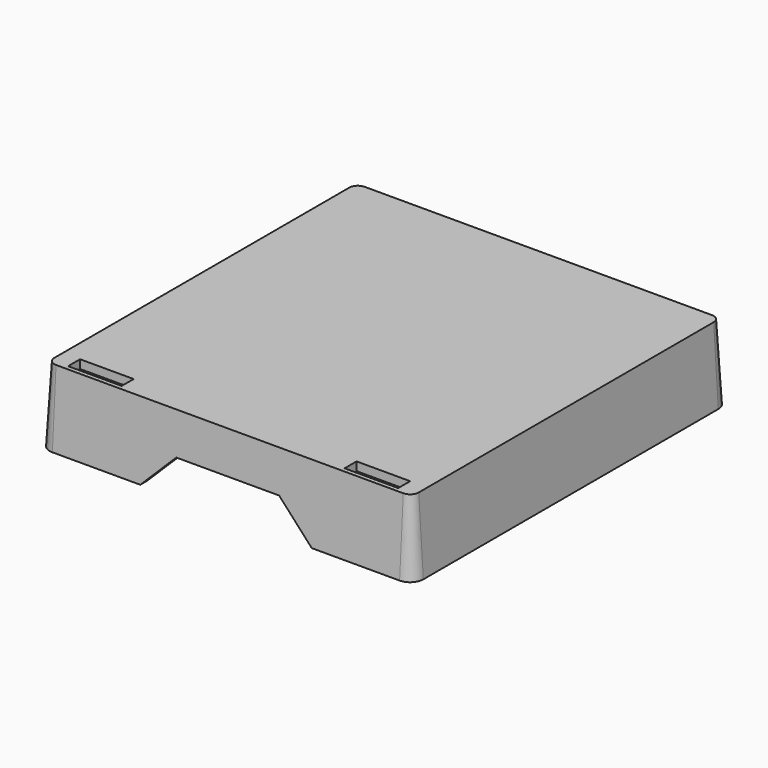
from build123d import *

# Parameters (mm, degrees)
F1_DEPTH  = 17.5
F1_TAPER  = -3.5
F3_DEPTH  = 75
F4_T      = 2
F5_W      = 12.5
F5_H      = 3.5
F6_DEPTH  = 17.5010001
F7_R      = 4
F8_DEPTH  = 31.5
F9_SIZE   = 3
F11_W     = 25
F11_H     = 20
F12_DEPTH = 10


# Not quite as in the source:
# - a shell that OpenCascade refuses in one call is made with other operations: the cavity is built on its own and cut out


with BuildPart() as f1:
    # F0 (on Top) → F1 (new body)
    with BuildSketch(Plane.XY):
        with BuildLine():
            Line((-40.5, -45), (40.5, -45))
            ThreePointArc((40.5, -45), (41.9142135624, -44.4142135624), (42.5, -43))
            Line((42.5, -43), (42.5, 43))
            ThreePointArc((42.5, 43), (41.9142135624, 44.4142135624), (40.5, 45))
            Line((40.5, 45), (-40.5, 45))
            ThreePointArc((-40.5, 45), (-41.9142135624, 44.4142135624), (-42.5, 43))
            Line((-42.5, 43), (-42.5, -43))
            ThreePointArc((-42.5, -43), (-41.9142135624, -44.4142135624), (-40.5, -45))
        make_face()
    extrude(amount=-F1_DEPTH, taper=F1_TAPER)

    # F2 (on Front) → F3 (cut, symmetric)
    with BuildSketch(Plane.XZ):
        Polygon((-20, -17.5), (0, -17.5), (20, -17.5), (12, -9.5), (0, -9.5), (-12, -9.5), align=None)
    extrude(amount=F3_DEPTH, both=True, mode=Mode.SUBTRACT)

    # F4: shell of thickness 2, made by hand


with BuildPart() as f4_core1:
    # F4_t2: copy of F1
    add(f1.part)

    # the walls: a layer under each face that stays
    f4_faces = [f4_core1.faces().sort_by_distance(p)[0] for p in [
        (0, -45.5351729263, -8.75),
        (-42.2926379677, -44.7926379677, -8.75),
        (42.2926379677, -44.7926379677, -8.75),
        (0, 0, 0),
        (-43.0351729263, 0, -8.75),
        (-42.2926379677, 44.7926379677, -8.75),
        (0, 45.5351729263, -8.75),
        (42.2926379677, 44.7926379677, -8.75),
        (43.0351729263, 0, -8.75),
    ]]
    thicken(f4_faces, amount=-F4_T, mode=Mode.SUBTRACT)


with BuildPart() as f1_1:
    add(f1.part)

    # what is left inside the walls is the cavity
    f4_cavity = [f4_core1.part.solids().sort_by_distance(p)[0] for p in [
        (-13.539529, 0, -2.02),
    ]]
    add(f4_cavity, mode=Mode.SUBTRACT)

    # F5 (on Top) → F6 (cut, through all)
    with BuildSketch(Plane.XY):
        with Locations((-32.25, -42.25)):
            Rectangle(F5_W, F5_H)
        with Locations((32.25, -42.25)):
            Rectangle(F5_W, F5_H)
    extrude(amount=-F6_DEPTH, mode=Mode.SUBTRACT)

    # F7 (on Top) → F8 (join)
    with BuildSketch(Plane.XY):
        with Locations((-17, -6)):
            Circle(F7_R)
        with Locations((17, -6)):
            Circle(F7_R)
    extrude(amount=-F8_DEPTH)

    # F9
    f9_edges = [f1_1.edges().sort_by_distance(p)[0] for p in [
        (-21, -6, -31.5),
        (13, -6, -31.5),
    ]]
    chamfer(f9_edges, length=F9_SIZE)

    # F11 (on offset) → F12 (join)
    with BuildSketch(Plane(origin=(0, 0, -23.5), x_dir=(1, 0, 0), z_dir=(0, 0, -1))):
        with Locations((-13, 6)):
            Rectangle(F11_W, F11_H)
        with Locations((13, 6)):
            Rectangle(F11_W, F11_H)
    extrude(amount=-F12_DEPTH)


solid = f1_1.part
